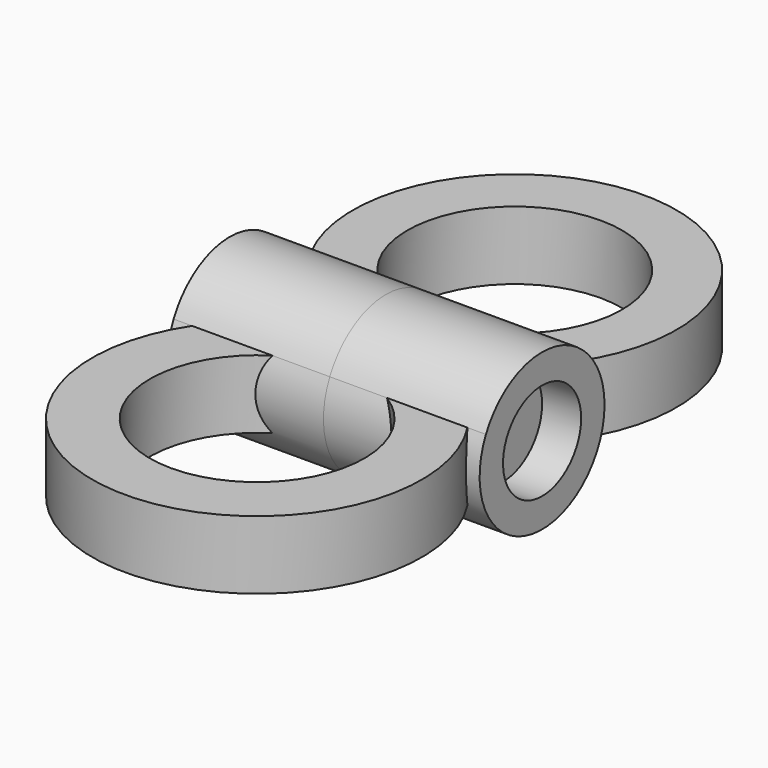
from build123d import *

# Parameters (mm, degrees)
F0_R          = 11
F1_DEPTH      = 7
F3_DEPTH      = 16
F3_DEPTH_BACK = 16
F4_R          = 5
F5_DEPTH      = 4
F6_R          = 5
F7_DEPTH      = 4


# Not quite as in the source:
# - a feature of the source that left no trace in its solid (it failed there, or was rolled back) is left out


with BuildPart() as f1:
    # F0 (on Top) → F1 (new body)
    with BuildSketch(Plane.XY):
        with BuildLine():
            ThreePointArc((13.2046790968, 10.5469991105), (14.5476279215, 16.7175814785), (13.1493192392, 22.8758548676))
            ThreePointArc((13.1493192392, 22.8758548676), (0, 49.5952677326), (-13.1493192392, 22.8758548676))
            ThreePointArc((-13.1493192392, 22.8758548676), (-14.5476279215, 16.7175814785), (-13.2046790968, 10.5469991105))
            ThreePointArc((-13.2046790968, 10.5469991105), (0, -16.8997852142), (13.2046790968, 10.5469991105))
        make_face()
        Circle(F0_R, mode=Mode.SUBTRACT)
        with Locations((0, 33)):
            Circle(F0_R, mode=Mode.SUBTRACT)
    extrude(amount=F1_DEPTH)

    # F2 (on Right) → F3 (join, two sides)
    with BuildSketch(Plane.YZ) as f3_sk:
        with BuildLine():
            ThreePointArc((9.306252715, 7), (14.7041684767, -4.2958315233), (24.5, 3.5))
            ThreePointArc((24.5, 3.5), (18.2958315233, 11.2958315233), (9.306252715, 7))
        make_face()
    extrude(amount=F3_DEPTH)
    extrude(f3_sk.sketch, amount=-F3_DEPTH_BACK)

    # F4 (on face) → F5 (cut)
    with BuildSketch(Plane.YZ.offset(16)):
        with Locations((16.5, 3.5)):
            Circle(F4_R)
    extrude(amount=-F5_DEPTH, mode=Mode.SUBTRACT)

    # F6 (on face) → F7 (cut)
    with BuildSketch(Plane(origin=(-16, 0, 0), x_dir=(0, -1, 0), z_dir=(-1, 0, 0))):
        with Locations((-16.5, 3.5)):
            Circle(F6_R)
    extrude(amount=-F7_DEPTH, mode=Mode.SUBTRACT)


solid = f1.part
